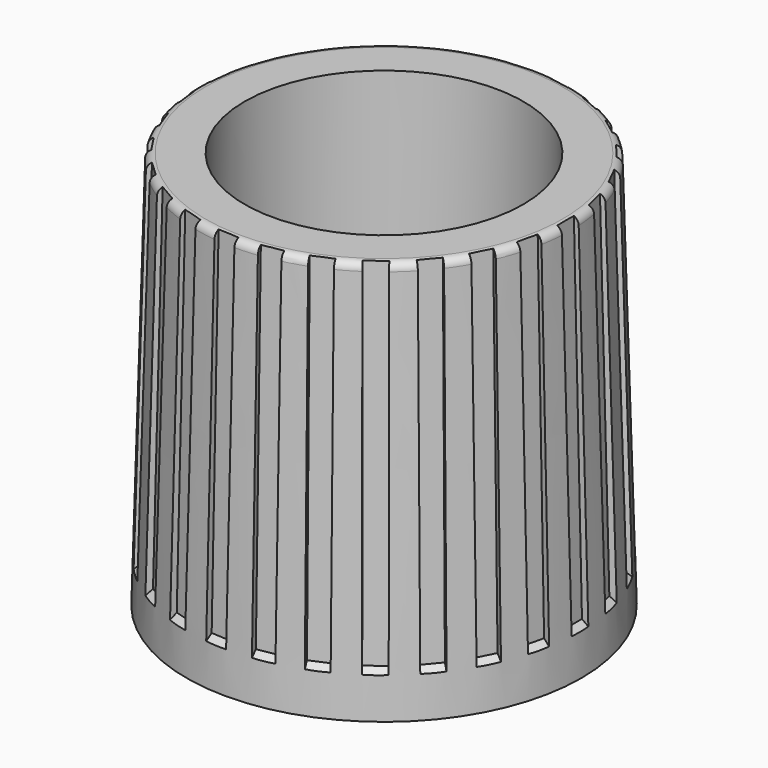
from build123d import *

# Parameters (mm, degrees)
F3_DEPTH        = 0.4
F3_COPIES_COUNT = 27
F3_COPIES_ANGLE = 346.58


# Not quite as in the source:
# - a pattern or mirror of a feature is missing from the dataset's text; its kind, count and spacing are read off the source's solid


with BuildPart() as f1:
    # F0 (on Front) → F1 (revolve)
    with BuildSketch(Plane.XZ):
        with BuildLine():
            Line((-5.65, 8.28), (-5.33, 8.28))
            Line((-5.33, 8.28), (-5.33, 15.23))
            Line((-5.33, 15.23), (-6.8381590919, 15.23))
            ThreePointArc((-6.8381590919, 15.23), (-7.0473468063, 15.1450360439), (-7.138045082, 14.938270001))
            Line((-7.138045082, 14.938270001), (-7.55, 0))
            Line((-7.55, 0), (-5.65, 0))
            Line((-5.65, 0), (-5.65, 8.28))
        make_face()
    revolve(axis=Axis((0, 0, 7.6919164343), (0, 0, -1)))

    # F2 (on Front) → F3 (cut, symmetric)
    with BuildSketch(Plane.XZ):
        Polygon((9.3553589453, 15.256884048), (6.9424775429, 15.23), (7.2524495509, 1.7335590857), (9.3553589453, 0.1806417477), align=None)
    f3 = extrude(amount=F3_DEPTH, both=True, mode=Mode.SUBTRACT)

    # F3_copies: F3 ×27 about axis
    f3_copies_axis = Axis((0, 0, 0), (0, 0, -1))
    for i in range(1, F3_COPIES_COUNT):
        add(f3.rotate(f3_copies_axis, i * F3_COPIES_ANGLE / (F3_COPIES_COUNT - 1)), mode=Mode.SUBTRACT)


solid = f1.part
